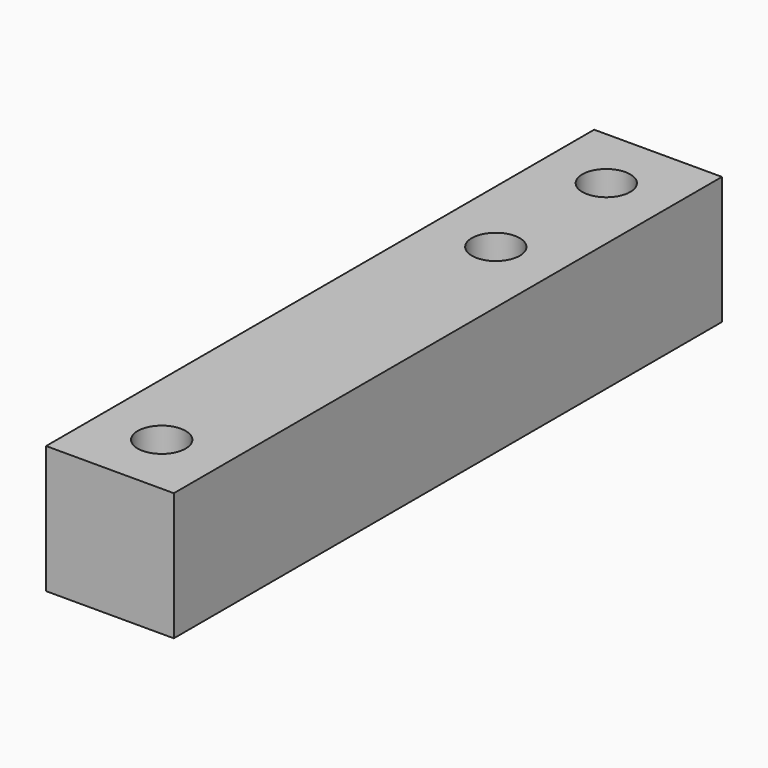
from build123d import *

# Parameters (mm, degrees)
F5_W     = 16
F5_H     = 16
F6_DEPTH = 42.9
F0_R     = 3
F7_DEPTH = 12.5
F2_SIZE  = 4.99999
F3_R     = 3
F4_DEPTH = 16.001


# Not quite as in the source:
# - a fillet or chamfer is up to 0.001 mm smaller than in the source, because OpenCascade refuses the exact size


with BuildPart() as f6:
    # F5 (on Front) → F6 (new body, symmetric)
    with BuildSketch(Plane.XZ):
        Rectangle(F5_W, F5_H)
    extrude(amount=F6_DEPTH, both=True)

    # F0 (on Top) → F7 (cut, symmetric)
    with BuildSketch(Plane.XY):
        with Locations((0, -34.8)):
            Circle(F0_R)
        with Locations((0, 34.8)):
            Circle(F0_R)
    extrude(amount=F7_DEPTH, both=True, mode=Mode.SUBTRACT)

    # F2 (size 5 in the source; OpenCascade refuses exactly that, so slightly less here)
    f2_edges = [f6.edges().sort_by_distance(p)[0] for p in [
        (-3, 34.8, -8),
    ]]
    chamfer(f2_edges, length=F2_SIZE)

    # F3 (on face) → F4 (cut, through all)
    with BuildSketch(Plane.XY.offset(8)):
        with Locations((0, 17.5)):
            Circle(F3_R)
    extrude(amount=-F4_DEPTH, mode=Mode.SUBTRACT)


solid = f6.part
